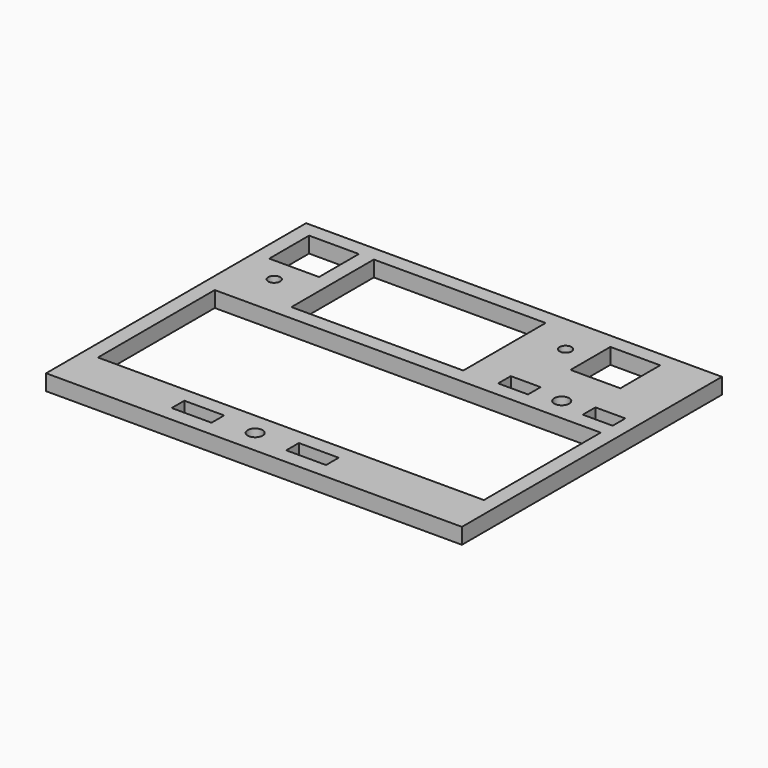
from build123d import *

# Parameters (mm, degrees)
F0_W     = 83.5
F0_H     = 65.2625
F0_W_2   = 8
F0_H_2   = 3.175
F0_W_3   = 77.5
F0_H_3   = 29.325
F0_W_4   = 34.5
F0_H_4   = 20.675
F0_W_5   = 6
F0_W_6   = 10
F0_H_5   = 10
F0_R     = 1.2
F1_DEPTH = 3.175


# Not quite as in the source:
# - a length typed as a fraction of an inch, garbled in the dataset ("3 / 203.2 mm" for 3/8 in), is restored
# - a feature names something its author has since deleted; it is built from what else it names


with BuildPart() as f1:
    # F0 (on Top) → F1 (new body)
    with BuildSketch(Plane.XY):
        with Locations((-5.970182175, 24.7772044539)):
            Rectangle(F0_W, F0_H)
        with Locations((-20.970182175, -3.1790455461)):
            Rectangle(F0_W_2, F0_H_2, mode=Mode.SUBTRACT)
        with BuildLine():
            ThreePointArc((-9.470182175, -4.6790455461), (-10.5308423468, -2.1183853743), (-7.970182175, -3.1790455461))
            ThreePointArc((-7.970182175, -3.1790455461), (-8.4095220032, -4.2397057179), (-9.470182175, -4.6790455461))
        make_face(mode=Mode.SUBTRACT)
        with Locations((2.029817825, -3.1790455461)):
            Rectangle(F0_W_2, F0_H_2, mode=Mode.SUBTRACT)
        with Locations((-5.970182175, 16.0709544539)):
            Rectangle(F0_W_3, F0_H_3, mode=Mode.SUBTRACT)
        Polygon((-44.720182175, 34.4084544539), (-44.720182175, 44.4084544539), (-44.720182175, 54.4084544539), (-34.720182175, 54.4084544539), (-34.720182175, 44.4084544539), (-34.720182175, 34.4084544539), align=None, mode=Mode.SUBTRACT)
        with Locations((-14.470182175, 44.0709544539)):
            Rectangle(F0_W_4, F0_H_4, mode=Mode.SUBTRACT)
        with Locations((12.779817825, 35.3209544539)):
            Rectangle(F0_W_5, F0_H_2, mode=Mode.SUBTRACT)
        with BuildLine():
            ThreePointArc((21.279817825, 33.8209544539), (20.2191576532, 36.3816146257), (22.779817825, 35.3209544539))
            ThreePointArc((22.779817825, 35.3209544539), (22.3404779968, 34.2602942821), (21.279817825, 33.8209544539))
        make_face(mode=Mode.SUBTRACT)
        with Locations((29.779817825, 35.3209544539)):
            Rectangle(F0_W_5, F0_H_2, mode=Mode.SUBTRACT)
        Polygon((25.779817825, 44.4084544539), (15.779817825, 44.4084544539), (5.779817825, 44.4084544539), (5.779817825, 54.4084544539), (15.779817825, 54.4084544539), (25.779817825, 54.4084544539), align=None, mode=Mode.SUBTRACT)
        with Locations((-39.720182175, 39.4084544539)):
            Rectangle(F0_W_6, F0_H_5)
        with Locations((-39.720182175, 39.4084544539)):
            Circle(F0_R, mode=Mode.SUBTRACT)
        with Locations((10.779817825, 49.4084544539)):
            Rectangle(F0_W_6, F0_H_5)
        with Locations((10.779817825, 49.4084544539)):
            Circle(F0_R, mode=Mode.SUBTRACT)
    extrude(amount=F1_DEPTH)


solid = f1.part
